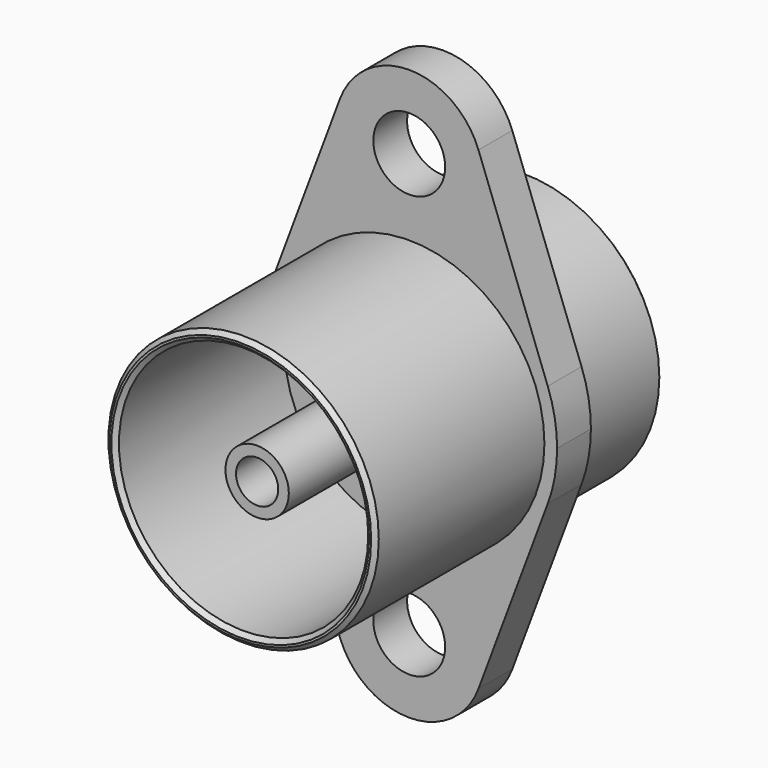
from build123d import *

# Parameters (mm, degrees)
F0_R     = 1.7
F0_R_2   = 6.4
F0_R_3   = 5.9
F0_R_4   = 1.5
F0_R_5   = 1
F1_DEPTH = 2
F2_DEPTH = 7
F3_DEPTH = 10
F4_DEPTH = 9
F6_SIZE  = 0.2


# Not quite as in the source:
# - the program builds the solid bodies; features that only make, move or delete a surface that nothing else refers to are left out


with BuildPart() as f1:
    # F0 (on Front) → F1 (new body)
    with BuildSketch(Plane.XZ):
        with BuildLine():
            Line((6.5572478983, 2.45), (3.2786239492, 11.225))
            ThreePointArc((3.2786239492, 11.225), (0, 13.5), (-3.2786239492, 11.225))
            Line((-3.2786239492, 11.225), (-6.5572478983, 2.45))
            ThreePointArc((-6.5572478983, 2.45), (0, 7), (6.5572478983, 2.45))
        make_face()
        with Locations((0, 10)):
            Circle(F0_R, mode=Mode.SUBTRACT)
        with BuildLine():
            ThreePointArc((6.5572478983, -2.45), (0, -7), (-6.5572478983, -2.45))
            Line((-6.5572478983, -2.45), (-3.2786239492, -11.225))
            ThreePointArc((-3.2786239492, -11.225), (0, -13.5), (3.2786239492, -11.225))
            Line((3.2786239492, -11.225), (6.5572478983, -2.45))
        make_face()
        with Locations((0, -10)):
            Circle(F0_R, mode=Mode.SUBTRACT)
        with BuildLine():
            ThreePointArc((7, 0), (6.8884227254, 1.2448423016), (6.5572478983, 2.45))
            ThreePointArc((6.5572478983, 2.45), (0, 7), (-6.5572478983, 2.45))
            ThreePointArc((-6.5572478983, 2.45), (-7, 0), (-6.5572478983, -2.45))
            ThreePointArc((-6.5572478983, -2.45), (0, -7), (6.5572478983, -2.45))
            ThreePointArc((6.5572478983, -2.45), (6.8884227254, -1.2448423016), (7, 0))
        make_face()
        Circle(F0_R_2, mode=Mode.SUBTRACT)
        Circle(F0_R_2)
        Circle(F0_R_3, mode=Mode.SUBTRACT)
        Circle(F0_R_3)
        Circle(F0_R_4, mode=Mode.SUBTRACT)
        Circle(F0_R_4)
        Circle(F0_R_5, mode=Mode.SUBTRACT)
        Circle(F0_R_5)
    extrude(amount=-F1_DEPTH)

    # F0 (on Front) → F2 (join)
    with BuildSketch(Plane.XZ):
        Circle(F0_R_2)
        Circle(F0_R_3, mode=Mode.SUBTRACT)
        Circle(F0_R_3)
        Circle(F0_R_4, mode=Mode.SUBTRACT)
        Circle(F0_R_4)
        Circle(F0_R_5, mode=Mode.SUBTRACT)
        Circle(F0_R_5)
    extrude(amount=-F2_DEPTH)

    # F0 (on Front) → F3 (join)
    with BuildSketch(Plane.XZ):
        Circle(F0_R_2)
        Circle(F0_R_3, mode=Mode.SUBTRACT)
    extrude(amount=F3_DEPTH)

    # F0 (on Front) → F4 (join)
    with BuildSketch(Plane.XZ):
        Circle(F0_R_4)
        Circle(F0_R_5, mode=Mode.SUBTRACT)
    extrude(amount=F4_DEPTH)

    # F6
    f6_edges = [f1.edges().sort_by_distance(p)[0] for p in [
        (-6.4, -10, 0),
        (-5.9, -10, 0),
        (-6.4, 7, 0),
    ]]
    chamfer(f6_edges, length=F6_SIZE)


solid = f1.part
